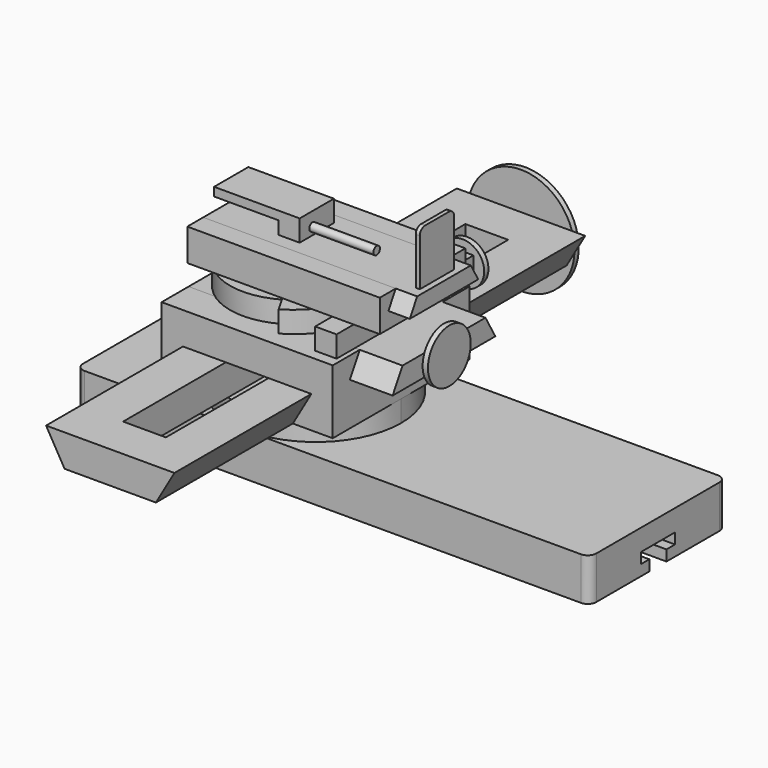
from build123d import *

# Parameters (mm, degrees)
F0_W           = 304.8
F0_H           = 101.6
F1_DEPTH       = 25.4
F2_R           = 5.08
F4_DEPTH       = 304.801
F6_DEPTH       = 12.7
F7_W           = 101.6
F7_H           = 101.6
F8_DEPTH       = 38.1
F10_DEPTH      = 101.6
F12_DEPTH      = 101.6
F13_DEPTH      = 101.6
F14_DEPTH      = 203.2
F15_W          = 25.4
F15_H          = 254
F16_DEPTH      = 19.05
F17_R          = 31.75
F18_DEPTH      = 3.175
F19_DEPTH      = 101.6
F19_DEPTH_BACK = 25.4
F20_R          = 15.875
F21_DEPTH      = 3.175
F23_DEPTH      = 12.7
F24_W          = 12.7
F24_H          = 101.6
F25_DEPTH      = 12.7
F26_R          = 12.7
F27_DEPTH      = 3.175
F28_W          = 114.3
F28_H          = 63.5
F29_DEPTH      = 19.05
F31_DEPTH      = 114.3
F32_DEPTH      = 127
F33_W          = 50.8
F33_H          = 25.4
F34_DEPTH      = 12.7
F35_W          = 12.7
F35_H          = 7.62
F36_DEPTH      = 38.1
F37_R          = 2.413
F38_DEPTH      = 12.7
F39_DEPTH      = 3.175
F39_DEPTH_BACK = 50.8
F40_W          = 2.38125
F40_H          = 25.4
F41_DEPTH      = 31.75
F42_R          = 3.81


with BuildPart() as f1:
    # F0 (on Top) → F1 (new body)
    with BuildSketch(Plane.XY):
        with Locations((152.4, 50.8)):
            Rectangle(F0_W, F0_H)
    extrude(amount=F1_DEPTH)

    # F2
    f2_edges = [f1.edges().sort_by_distance(p)[0] for p in [
        (0, 0, 12.7),
        (304.8, 0, 12.7),
        (304.8, 101.6, 12.7),
        (0, 101.6, 12.7),
    ]]
    fillet(f2_edges, radius=F2_R)

    # F3 (on face) → F4 (cut, through all)
    with BuildSketch(Plane.YZ.offset(304.8)):
        Polygon((44.45, 6.35), (44.45, 0), (57.15, 0), (57.15, 6.35), (63.5, 6.35), (63.5, 12.7), (38.1, 12.7), (38.1, 6.35), align=None)
    extrude(amount=-F4_DEPTH, mode=Mode.SUBTRACT)


with BuildPart() as f6:
    # F5 (on face) → F6 (new body)
    with BuildSketch(Plane.XY.offset(25.4)):
        with BuildLine():
            ThreePointArc((101.6, 0), (137.5210244843, 14.8789755157), (152.4, 50.8))
            ThreePointArc((152.4, 50.8), (137.5210244843, 86.7210244843), (101.6, 101.6))
            ThreePointArc((101.6, 101.6), (50.8, 50.8), (101.6, 0))
        make_face()
    extrude(amount=F6_DEPTH)


with BuildPart() as f8:
    # F7 (on face) → F8 (new body)
    with BuildSketch(Plane.XY.offset(38.1)):
        with Locations((101.6, 50.8)):
            Rectangle(F7_W, F7_H)
    extrude(amount=F8_DEPTH)

    # F9 (on face) → F10 (cut, through all)
    with BuildSketch(Plane.XZ):
        Polygon((63.5, 57.15), (74.4985226281, 38.1), (128.7014773719, 38.1), (139.7, 57.15), align=None)
    extrude(amount=-F10_DEPTH, mode=Mode.SUBTRACT)

    # F11 (on face) → F12 (cut, through all)
    with BuildSketch(Plane.YZ.offset(152.4)):
        Polygon((81.5676515813, 76.2), (20.0323484187, 76.2), (12.7, 63.5), (88.9, 63.5), align=None)
    extrude(amount=-F12_DEPTH, mode=Mode.SUBTRACT)


with BuildPart() as f13:
    # F9 (on face) → F13 (new body)
    with BuildSketch(Plane.XZ):
        Polygon((63.5, 57.15), (74.4985226281, 38.1), (128.7014773719, 38.1), (139.7, 57.15), align=None)
    extrude(amount=F13_DEPTH)

    # F9 (on face) → F14 (join)
    with BuildSketch(Plane.XZ):
        Polygon((63.5, 57.15), (74.4985226281, 38.1), (128.7014773719, 38.1), (139.7, 57.15), align=None)
    extrude(amount=-F14_DEPTH)

    # F15 (on face) → F16 (cut, through all)
    with BuildSketch(Plane.XY.offset(57.15)):
        with Locations((101.6, 50.8)):
            Rectangle(F15_W, F15_H)
    extrude(amount=-F16_DEPTH, mode=Mode.SUBTRACT)


with BuildPart() as f18:
    # F17 (on face) → F18 (new body)
    with BuildSketch(Plane(origin=(0, 203.2, 0), x_dir=(-1, 0, 0), z_dir=(0, 1, 0))):
        with Locations((-101.6, 47.625)):
            Circle(F17_R)
    extrude(amount=F18_DEPTH)


with BuildPart() as f19:
    # F11 (on face) → F19 (new body, two sides)
    with BuildSketch(Plane.YZ.offset(152.4)) as f19_sk:
        Polygon((81.5676515813, 76.2), (20.0323484187, 76.2), (12.7, 63.5), (88.9, 63.5), align=None)
    extrude(amount=-F19_DEPTH)
    extrude(f19_sk.sketch, amount=F19_DEPTH_BACK)


with BuildPart() as f21:
    # F20 (on face) → F21 (new body)
    with BuildSketch(Plane.YZ.offset(177.8)):
        with Locations((50.8, 69.85)):
            Circle(F20_R)
    extrude(amount=F21_DEPTH)


with BuildPart() as f23:
    # F22 (on face) → F23 (new body)
    with BuildSketch(Plane.XY.offset(76.2)):
        with BuildLine():
            Line((112.893734675, 92.3583675204), (107.95, 83.7955678842))
            ThreePointArc((107.95, 83.7955678842), (50.8, 50.8), (107.95, 17.8044321158))
            Line((107.95, 17.8044321158), (112.893734675, 9.2416324796))
            ThreePointArc((112.893734675, 9.2416324796), (136.8874693499, 50.8), (112.893734675, 92.3583675204))
        make_face()
    extrude(amount=F23_DEPTH)


with BuildPart() as f25:
    # F24 (on face) → F25 (new body)
    with BuildSketch(Plane.XY.offset(76.2)):
        with Locations((143.2374693499, 57.15)):
            Rectangle(F24_W, F24_H)
    extrude(amount=F25_DEPTH)


with BuildPart() as f27:
    # F26 (on face) → F27 (new body)
    with BuildSketch(Plane(origin=(0, 107.95, 0), x_dir=(-1, 0, 0), z_dir=(0, 1, 0))):
        with Locations((-143.2374693499, 82.55)):
            Circle(F26_R)
    extrude(amount=F27_DEPTH)


with BuildPart() as f29:
    # F28 (on face) → F29 (new body)
    with BuildSketch(Plane.XY.offset(88.9)):
        with Locations((107.95, 50.8)):
            Rectangle(F28_W, F28_H)
    extrude(amount=F29_DEPTH)

    # F30 (on face) → F31 (cut, through all)
    with BuildSketch(Plane(origin=(50.8, 0, 0), x_dir=(0, -1, 0), z_dir=(-1, 0, 0))):
        Polygon((-30.899261314, 107.95), (-70.700738686, 107.95), (-76.2, 98.425), (-25.4, 98.425), align=None)
    extrude(amount=-F31_DEPTH, mode=Mode.SUBTRACT)


with BuildPart() as f32:
    # F30 (on face) → F32 (new body)
    with BuildSketch(Plane(origin=(50.8, 0, 0), x_dir=(0, -1, 0), z_dir=(-1, 0, 0))):
        Polygon((-30.899261314, 107.95), (-70.700738686, 107.95), (-76.2, 98.425), (-25.4, 98.425), align=None)
    extrude(amount=-F32_DEPTH)


with BuildPart() as f34:
    # F33 (on face) → F34 (new body)
    with BuildSketch(Plane.XY.offset(107.95)):
        with Locations((76.2, 51.650738686)):
            Rectangle(F33_W, F33_H)
    extrude(amount=F34_DEPTH)

    # F35 (on face) → F36 (cut)
    with BuildSketch(Plane(origin=(50.8, 0, 0), x_dir=(0, -1, 0), z_dir=(-1, 0, 0))):
        with Locations((-45.300738686, 111.76)):
            Rectangle(F35_W, F35_H)
    extrude(amount=-F36_DEPTH, mode=Mode.SUBTRACT)

    # F37 (on face) → F38 (cut, through all)
    with BuildSketch(Plane(origin=(88.9, 0, 0), x_dir=(0, -1, 0), z_dir=(-1, 0, 0))):
        with Locations((-48.475738686, 112.395)):
            Circle(F37_R)
    extrude(amount=-F38_DEPTH, mode=Mode.SUBTRACT)


with BuildPart() as f39:
    # F37 (on face) → F39 (new body, two sides)
    with BuildSketch(Plane(origin=(88.9, 0, 0), x_dir=(0, -1, 0), z_dir=(-1, 0, 0))) as f39_sk:
        with Locations((-48.475738686, 112.395)):
            Circle(F37_R)
    extrude(amount=F39_DEPTH)
    extrude(f39_sk.sketch, amount=-F39_DEPTH_BACK)


with BuildPart() as f41:
    # F40 (on face) → F41 (new body)
    with BuildSketch(Plane.XY.offset(107.95)):
        with Locations((173.1103308957, 49.949261314)):
            Rectangle(F40_W, F40_H)
    extrude(amount=F41_DEPTH)

    # F42
    f42_edges = [f41.edges().sort_by_distance(p)[0] for p in [
        (173.110331, 37.249261, 139.7),
        (173.110331, 62.649261, 139.7),
    ]]
    fillet(f42_edges, radius=F42_R)


solid = Compound([f1.part, f6.part, f8.part, f13.part, f18.part, f19.part, f21.part, f23.part, f25.part, f27.part, f29.part, f32.part, f34.part, f39.part, f41.part])
